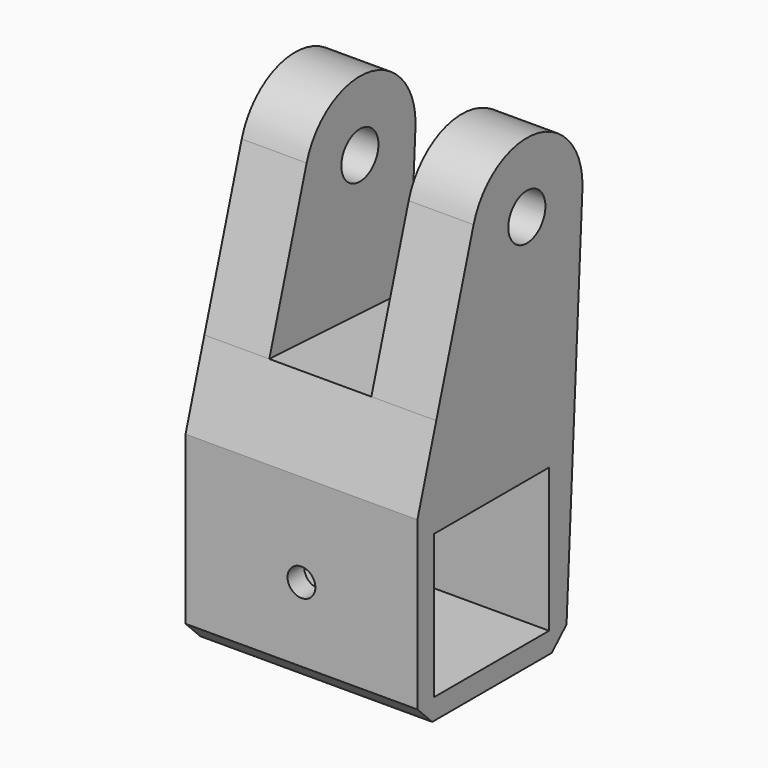
from build123d import *

# Parameters (mm, degrees)
F0_R        = 2.5
F0_W        = 20
F0_H        = 20
F0_W_2      = 15.5
F0_H_2      = 15.5
F1_DEPTH    = 25
F2_START    = -7
F2_DEPTH    = 11
F3_R        = 1.5
F4_DEPTH    = 25
F5_T1_DEPTH = 35.2867319519
F5_T3_DEPTH = 34.7792924718


# Not quite as in the source:
# - a fillet or chamfer that OpenCascade refuses, or shapes differently, is made with other operations: its cross-section is extruded or revolved along the edge and cut away or added


with BuildPart() as f1:
    # F0 (on Right) → F1 (new body)
    with BuildSketch(Plane.YZ):
        Polygon((-55.5157013459, 38.3205534184), (-58.0598865449, 29.9461055547), (-38.0598865449, 29.9461055547), (-38.0598865449, 9.9461055547), (-36.6123928978, 37.3210094949), align=None)
        with BuildLine():
            ThreePointArc((-35.8098865449, 52.6961055547), (-42.207857033, 60.1146991515), (-50.4860281329, 54.8762413095))
            ThreePointArc((-50.4860281329, 54.8762413095), (-44.6074616185, 45.3092050593), (-35.8203493916, 52.3000838016))
            ThreePointArc((-35.8203493916, 52.3000838016), (-35.8125027129, 52.4980255834), (-35.8098865449, 52.6961055547))
        make_face()
        with Locations((-43.3098865449, 52.6961055547)):
            Circle(F0_R, mode=Mode.SUBTRACT)
        with Locations((-48.0598865449, 19.9461055547)):
            Rectangle(F0_W, F0_H)
        with Locations((-48.0598865449, 19.9461055547)):
            Rectangle(F0_W_2, F0_H_2, mode=Mode.SUBTRACT)
        with BuildLine():
            Line((-50.4860281329, 54.8762413095), (-55.5157013459, 38.3205534184))
            Line((-55.5157013459, 38.3205534184), (-36.6123928978, 37.3210094949))
            Line((-36.6123928978, 37.3210094949), (-35.8203493916, 52.3000838016))
            ThreePointArc((-35.8203493916, 52.3000838016), (-44.6074616185, 45.3092050593), (-50.4860281329, 54.8762413095))
        make_face()
    extrude(amount=-F1_DEPTH)

    # F0 (on Right) → F2 (cut)
    with BuildSketch(Plane.YZ.offset(F2_START)):
        with BuildLine():
            Line((-50.4860281329, 54.8762413095), (-55.5157013459, 38.3205534184))
            Line((-55.5157013459, 38.3205534184), (-36.6123928978, 37.3210094949))
            Line((-36.6123928978, 37.3210094949), (-35.8203493916, 52.3000838016))
            ThreePointArc((-35.8203493916, 52.3000838016), (-44.6074616185, 45.3092050593), (-50.4860281329, 54.8762413095))
        make_face()
        with BuildLine():
            ThreePointArc((-35.8098865449, 52.6961055547), (-42.207857033, 60.1146991515), (-50.4860281329, 54.8762413095))
            ThreePointArc((-50.4860281329, 54.8762413095), (-44.6074616185, 45.3092050593), (-35.8203493916, 52.3000838016))
            ThreePointArc((-35.8203493916, 52.3000838016), (-35.8125027129, 52.4980255834), (-35.8098865449, 52.6961055547))
        make_face()
        with Locations((-43.3098865449, 52.6961055547)):
            Circle(F0_R, mode=Mode.SUBTRACT)
    extrude(amount=-F2_DEPTH, mode=Mode.SUBTRACT)

    # F3 (on face) → F4 (cut)
    with BuildSketch(Plane.XZ.offset(58.0598865449)):
        with Locations((-12.5, 19.9461055547)):
            Circle(F3_R)
    extrude(amount=-F4_DEPTH, mode=Mode.SUBTRACT)

    # F5: chamfer of 2 on 2 edges, made by hand

    # F5_s2 → F5_t1 (cut)
    with BuildSketch(Plane.YZ.offset(-30.1433659759)):
        Polygon((-56.0598865449, 9.9461055547), (-58.0598865449, 11.9461055547), (-58.0598865449, 9.9461055547), align=None)
    extrude(amount=F5_T1_DEPTH, mode=Mode.SUBTRACT)

    # F5_s4 → F5_t3 (cut)
    with BuildSketch(Plane.YZ.offset(-29.8896462359)):
        Polygon((-37.959717296, 11.8404997539), (-39.9569272035, 9.9461055547), (-38.0598865449, 9.9461055547), align=None)
    extrude(amount=F5_T3_DEPTH, mode=Mode.SUBTRACT)


solid = f1.part
